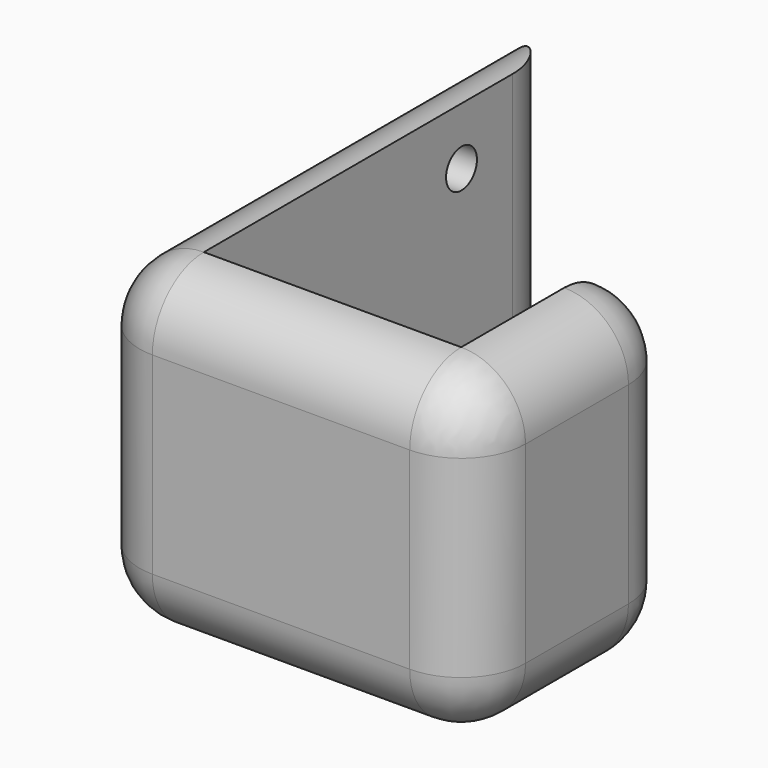
from build123d import *

# Parameters (mm, degrees)
F1_DEPTH    = 25
F2_R        = 4.99999
F3_T1_DEPTH = 40.00001
F3_T3_DEPTH = 45.00001
F3_T6_ANGLE = 90
F4_R        = 4.99999
F5_R        = 4.99999
F6_R        = 4.99999
F7_T1_DEPTH = 27.50001
F7_T3_DEPTH = 25.0000100044
F7_T6_ANGLE = 90
F7_T8_ANGLE = 233.2969892316
F9_R        = 1.5
F10_DEPTH   = 6
F11_DEPTH   = 6


# Not quite as in the source:
# - a fillet or chamfer that OpenCascade refuses, or shapes differently, is made with other operations: its cross-section is extruded or revolved along the edge and cut away or added
# - a fillet or chamfer is up to 0.001 mm smaller than in the source, because OpenCascade refuses the exact size


with BuildPart() as f1:
    # F0 (on Top) → F1 (new body)
    with BuildSketch(Plane.XY):
        Polygon((-55.5160288679, 43.4392371902), (-60.5160288679, 43.4392371902), (-60.5160288679, 3.4392371902), (-30.5160288679, 3.4392371902), (-30.5160288679, 23.4392371902), (-35.5160288679, 23.4392371902), (-35.5160288679, 8.4392371902), (-55.5160288679, 8.4392371902), align=None)
    extrude(amount=F1_DEPTH)

    # F2 (radius 5 in the source; OpenCascade refuses exactly that, so slightly less here)
    f2_edges = [f1.edges().sort_by_distance(p)[0] for p in [
        (-45.516029, 3.439237, 25),
    ]]
    fillet(f2_edges, radius=F2_R)

    # F3: fillet of radius 5 on 1 edges, made by hand

    # F3_s2 → F3_t1 (cut)
    with BuildSketch(Plane.XZ.offset(-35.9392371902)):
        with BuildLine():
            ThreePointArc((-35.5160288679, 25), (-31.980494962, 23.5355339059), (-30.5160288679, 20))
            Line((-30.5160288679, 20), (-30.5160288679, 25))
            Line((-30.5160288679, 25), (-35.5160288679, 25))
        make_face()
    extrude(amount=F3_T1_DEPTH, mode=Mode.SUBTRACT)

    # F3_s4 → F3_t3 (cut)
    with BuildSketch(Plane.XY.offset(-12.5)):
        with BuildLine():
            ThreePointArc((-35.5160288679, 3.4392371902), (-31.980494962, 4.9037032843), (-30.5160288679, 8.4392371902))
            Line((-30.5160288679, 8.4392371902), (-30.5160288679, 3.4392371902))
            Line((-30.5160288679, 3.4392371902), (-35.5160288679, 3.4392371902))
        make_face()
    extrude(amount=F3_T3_DEPTH, mode=Mode.SUBTRACT)

    # F3_s5 → F3_t6 (revolve, cut)
    with BuildSketch(Plane.XY.offset(20.00001)):
        with BuildLine():
            ThreePointArc((-35.5160288679, 3.4392371902), (-31.9804984975, 4.9036997488), (-30.5160288679, 8.4392271902))
            Line((-30.5160288679, 8.4392271902), (-30.5160288679, 3.4392371902))
            Line((-30.5160288679, 3.4392371902), (-35.5160288679, 3.4392371902))
        make_face()
    revolve(axis=Axis((-30.5160288679, 8.4392271902, 20.00001), (-1, 0, 0)), revolution_arc=F3_T6_ANGLE, mode=Mode.SUBTRACT)

    # F4 (radius 5 in the source; OpenCascade refuses exactly that, so slightly less here)
    f4_edges = [f1.edges().sort_by_distance(p)[0] for p in [
        (-30.516029, 15.939237, 0),
    ]]
    fillet(f4_edges, radius=F4_R)

    # F5 (radius 5 in the source; OpenCascade refuses exactly that, so slightly less here)
    f5_edges = [f1.edges().sort_by_distance(p)[0] for p in [
        (-60.516029, 25.939232, 25),
    ]]
    fillet(f5_edges, radius=F5_R)

    # F6 (radius 5 in the source; OpenCascade refuses exactly that, so slightly less here)
    f6_edges = [f1.edges().sort_by_distance(p)[0] for p in [
        (-55.516029, 43.439237, 12.5),
    ]]
    fillet(f6_edges, radius=F6_R)

    # F7: fillet of radius 5 on 4 edges, made by hand

    # F7_s2 → F7_t1 (cut)
    with BuildSketch(Plane.XY.offset(-7.50001)):
        with BuildLine():
            ThreePointArc((-35.5160288679, 23.4392371902), (-31.980494962, 21.9747710962), (-30.5160288679, 18.4392371902))
            Line((-30.5160288679, 18.4392371902), (-30.5160288679, 23.4392371902))
            Line((-30.5160288679, 23.4392371902), (-35.5160288679, 23.4392371902))
        make_face()
    extrude(amount=F7_T1_DEPTH, mode=Mode.SUBTRACT)

    # F7_s4 → F7_t3 (cut)
    with BuildSketch(Plane.YZ.offset(-48.0160288701)):
        with BuildLine():
            ThreePointArc((18.4392371902, 0), (21.9747710962, 1.4644660941), (23.4392371902, 5))
            Line((23.4392371902, 5), (23.4392371902, 0))
            Line((23.4392371902, 0), (18.4392371902, 0))
        make_face()
    extrude(amount=F7_T3_DEPTH, mode=Mode.SUBTRACT)

    # F7_s5 → F7_t6 (revolve, cut)
    with BuildSketch(Plane.YZ.offset(-35.5160188679)):
        with BuildLine():
            ThreePointArc((18.4392371902, 0), (21.9747675606, 1.4644625585), (23.4392371902, 4.99999))
            Line((23.4392371902, 4.99999), (23.4392371902, 0))
            Line((23.4392371902, 0), (18.4392371902, 0))
        make_face()
    revolve(axis=Axis((-35.5160188679, 23.4392371902, 4.99999), (0, -1, 0)), revolution_arc=F7_T6_ANGLE, mode=Mode.SUBTRACT)

    # F7_s7 → F7_t8 (revolve, cut)
    with BuildSketch(Plane(origin=(-32.4130099886, 0, 24.1625626894), x_dir=(0, 1, 0), z_dir=(0.8017442393, 0, -0.5976672777))):
        with BuildLine():
            ThreePointArc((23.4392371902, -5.1918835033), (21.9747710962, -8.7274174092), (18.4392371902, -10.1918835033))
            Line((18.4392371902, -10.1918835033), (23.4392371902, -10.1918835033))
            Line((23.4392371902, -10.1918835033), (23.4392371902, -5.1918835033))
        make_face()
    revolve(axis=Axis((-35.516028868, 23.4392371902, 19.9999999999), (0, 1, 0)), revolution_arc=F7_T8_ANGLE, mode=Mode.SUBTRACT)

    # F9 (on offset) → F10 (cut)
    with BuildSketch(Plane.YZ.offset(-55)):
        with Locations((33.4674492478, 20.548062399)):
            Circle(F9_R)
    extrude(amount=-F10_DEPTH, mode=Mode.SUBTRACT)

    # F9 (on offset) → F11 (cut)
    with BuildSketch(Plane.YZ.offset(-55)):
        with Locations((33.4674492478, 20.548062399)):
            Circle(F9_R)
        with Locations((34.116756171, 3.7890784442)):
            Circle(F9_R)
    extrude(amount=-F11_DEPTH, mode=Mode.SUBTRACT)


solid = f1.part
